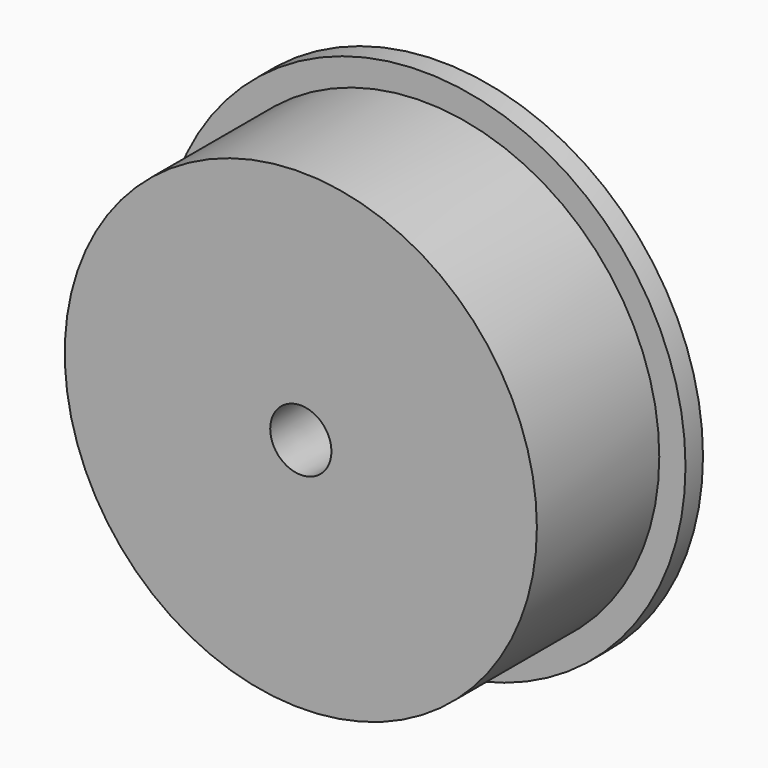
from build123d import *

# Parameters (mm, degrees)
F0_R     = 5.4
F1_DEPTH = 3.5
F2_R     = 6
F2_R_2   = 5.4
F3_DEPTH = 0.5
F4_R     = 4.75
F5_DEPTH = 3
F7_R     = 1.75
F8_DEPTH = 0.5
F9_R     = 0.75
F6_R     = 0.7


with BuildPart() as f1:
    # F0 (on Front) → F1 (new body)
    with BuildSketch(Plane.XZ):
        Circle(F0_R)
    extrude(amount=F1_DEPTH)

    # F2 (on face) → F3 (join)
    with BuildSketch(Plane(origin=(0, 0, 0), x_dir=(-1, 0, 0), z_dir=(0, 1, 0))):
        Circle(F2_R)
        Circle(F2_R_2, mode=Mode.SUBTRACT)
        Circle(F2_R_2)
    extrude(amount=F3_DEPTH)

    # F4 (on face) → F5 (cut)
    with BuildSketch(Plane(origin=(0, 0.5, 0), x_dir=(-1, 0, 0), z_dir=(0, 1, 0))):
        Circle(F4_R)
    extrude(amount=-F5_DEPTH, mode=Mode.SUBTRACT)

    # F7 (on face) → F8 (join)
    with BuildSketch(Plane(origin=(0, -2.5, 0), x_dir=(-1, 0, 0), z_dir=(0, 1, 0))):
        Circle(F7_R)
    extrude(amount=F8_DEPTH)

    # F9 (on face) → F10 section 0
    with BuildSketch(Plane(origin=(0, -2, 0), x_dir=(-1, 0, 0), z_dir=(0, 1, 0))):
        Circle(F9_R)
    # F6 (on face) → F10 section 1
    with BuildSketch(Plane.XZ.offset(3.5)):
        Circle(F6_R)
    loft(mode=Mode.SUBTRACT)


solid = f1.part
